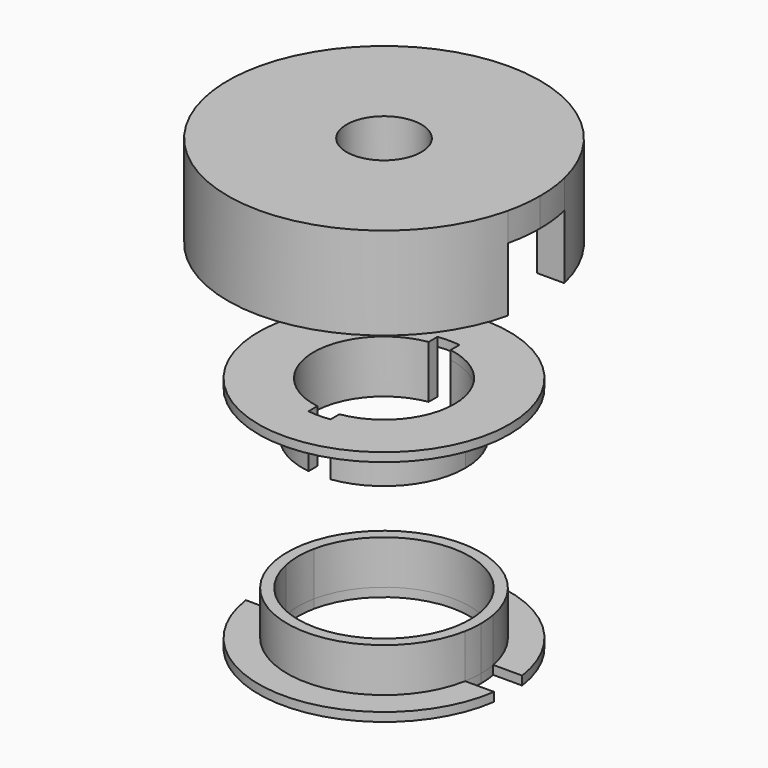
from build123d import *

# Parameters (mm, degrees)
F1_DEPTH  = 4.2
F0_R      = 3
F0_R_2    = 1.7
F2_DEPTH  = 1.3
F5_DEPTH  = 2
F4_R      = 5.7
F6_DEPTH  = 0.4
F7_DEPTH  = 2
F10_DEPTH = 2
F11_DEPTH = 0.4


with BuildPart() as f1:
    # F0 (on Top) → F1 (new body)
    with BuildSketch(Plane.XY):
        with BuildLine():
            Line((5.6789083458, 1.6), (6.9173694422, 1.6))
            ThreePointArc((6.9173694422, 1.6), (0, 7.1), (-6.9173694422, 1.6))
            Line((-6.9173694422, 1.6), (-5.6789083458, 1.6))
            ThreePointArc((-5.6789083458, 1.6), (0, 5.9), (5.6789083458, 1.6))
        make_face()
    extrude(amount=-F1_DEPTH)



with BuildPart() as f1b:
    # F0 (on Top) → F1, piece 2 (new body)
    with BuildSketch(Plane.XY):
        with BuildLine():
            ThreePointArc((-6.9173694422, -1.6), (0, -7.1), (6.9173694422, -1.6))
            Line((6.9173694422, -1.6), (5.6789083458, -1.6))
            ThreePointArc((5.6789083458, -1.6), (0, -5.9), (-5.6789083458, -1.6))
            Line((-5.6789083458, -1.6), (-6.9173694422, -1.6))
        make_face()
    extrude(amount=-F1_DEPTH)


with BuildPart() as f1c:
    # F0 (on Top) → F1, piece 3 (new body)
    with BuildSketch(Plane.XY):
        Circle(F0_R)
        Circle(F0_R_2, mode=Mode.SUBTRACT)
    extrude(amount=-F1_DEPTH)


with BuildPart() as f1_1:
    add(f1.part)

    add(f1b.part)  # F2 merges F1b

    add(f1c.part)  # F2 merges F1c
    # F0 (on Top) → F2 (join)
    with BuildSketch(Plane.XY):
        with BuildLine():
            Line((5.6789083458, 1.6), (6.9173694422, 1.6))
            ThreePointArc((6.9173694422, 1.6), (0, 7.1), (-6.9173694422, 1.6))
            Line((-6.9173694422, 1.6), (-5.6789083458, 1.6))
            ThreePointArc((-5.6789083458, 1.6), (0, 5.9), (5.6789083458, 1.6))
        make_face()
        with BuildLine():
            Line((-5.6789083458, 1.6), (-6.9173694422, 1.6))
            ThreePointArc((-6.9173694422, 1.6), (-7.1, 0), (-6.9173694422, -1.6))
            Line((-6.9173694422, -1.6), (-5.6789083458, -1.6))
            ThreePointArc((-5.6789083458, -1.6), (-5.9, 0), (-5.6789083458, 1.6))
        make_face()
        with BuildLine():
            ThreePointArc((-6.9173694422, -1.6), (0, -7.1), (6.9173694422, -1.6))
            Line((6.9173694422, -1.6), (5.6789083458, -1.6))
            ThreePointArc((5.6789083458, -1.6), (0, -5.9), (-5.6789083458, -1.6))
            Line((-5.6789083458, -1.6), (-6.9173694422, -1.6))
        make_face()
        with BuildLine():
            ThreePointArc((6.9173694422, -1.6), (7.0541946046, -0.8051946846), (7.1, 0))
            ThreePointArc((7.1, 0), (7.0541946046, 0.8051946846), (6.9173694422, 1.6))
            Line((6.9173694422, 1.6), (5.6789083458, 1.6))
            ThreePointArc((5.6789083458, 1.6), (5.8444657258, 0.807601622), (5.9, 0))
            ThreePointArc((5.9, 0), (5.8444657258, -0.807601622), (5.6789083458, -1.6))
            Line((5.6789083458, -1.6), (6.9173694422, -1.6))
        make_face()
        with BuildLine():
            Line((5.6789083458, -1.6), (5.6789083458, 1.6))
            ThreePointArc((5.6789083458, 1.6), (0, 5.9), (-5.6789083458, 1.6))
            Line((-5.6789083458, 1.6), (-5.6789083458, -1.6))
            ThreePointArc((-5.6789083458, -1.6), (0, -5.9), (5.6789083458, -1.6))
        make_face()
        Circle(F0_R, mode=Mode.SUBTRACT)
        with BuildLine():
            Line((-5.6789083458, -1.6), (-5.6789083458, 1.6))
            ThreePointArc((-5.6789083458, 1.6), (-5.9, 0), (-5.6789083458, -1.6))
        make_face()
        with BuildLine():
            ThreePointArc((5.9, 0), (5.8444657258, 0.807601622), (5.6789083458, 1.6))
            Line((5.6789083458, 1.6), (5.6789083458, -1.6))
            ThreePointArc((5.6789083458, -1.6), (5.8444657258, -0.807601622), (5.9, 0))
        make_face()
    extrude(amount=-F2_DEPTH)


with BuildPart() as f5:
    # F4 (on offset) → F5 (new body)
    with BuildSketch(Plane.XY.offset(-10)):
        with BuildLine():
            ThreePointArc((-0.5, 3.1606961259), (0, 3.2), (0.5, 3.1606961259))
            Line((0.5, 3.1606961259), (0.5, 3.666060556))
            ThreePointArc((0.5, 3.666060556), (0, 3.7), (-0.5, 3.666060556))
            Line((-0.5, 3.666060556), (-0.5, 3.1606961259))
        make_face()
        with BuildLine():
            ThreePointArc((-0.5, -3.1606961259), (-3.2, 0), (-0.5, 3.1606961259))
            Line((-0.5, 3.1606961259), (-0.5, 3.666060556))
            ThreePointArc((-0.5, 3.666060556), (-3.7, 0), (-0.5, -3.666060556))
            Line((-0.5, -3.666060556), (-0.5, -3.1606961259))
        make_face()
        with BuildLine():
            Line((0.5, -3.666060556), (0.5, -3.1606961259))
            ThreePointArc((0.5, -3.1606961259), (0, -3.2), (-0.5, -3.1606961259))
            Line((-0.5, -3.1606961259), (-0.5, -3.666060556))
            ThreePointArc((-0.5, -3.666060556), (0, -3.7), (0.5, -3.666060556))
        make_face()
        with BuildLine():
            ThreePointArc((0.5, 3.1606961259), (2.4331050121, 2.0784609691), (3.2, 0))
            ThreePointArc((3.2, 0), (2.4331050121, -2.0784609691), (0.5, -3.1606961259))
            Line((0.5, -3.1606961259), (0.5, -3.666060556))
            ThreePointArc((0.5, -3.666060556), (2.787471973, -2.4331050121), (3.7, 0))
            ThreePointArc((3.7, 0), (2.787471973, 2.4331050121), (0.5, 3.666060556))
            Line((0.5, 3.666060556), (0.5, 3.1606961259))
        make_face()
    extrude(amount=-F5_DEPTH)

    # F4 (on offset) → F6 (join)
    with BuildSketch(Plane.XY.offset(-10)):
        Circle(F4_R)
        with BuildLine():
            Line((0.5, 4.331942182), (0.5, 3.666060556))
            ThreePointArc((0.5, 3.666060556), (2.787471973, 2.4331050121), (3.7, 0))
            ThreePointArc((3.7, 0), (2.787471973, -2.4331050121), (0.5, -3.666060556))
            Line((0.5, -3.666060556), (0.5, -4.331942182))
            Line((0.5, -4.331942182), (-0.5, -4.331942182))
            Line((-0.5, -4.331942182), (-0.5, -3.666060556))
            ThreePointArc((-0.5, -3.666060556), (-3.7, 0), (-0.5, 3.666060556))
            Line((-0.5, 3.666060556), (-0.5, 4.331942182))
            Line((-0.5, 4.331942182), (0.5, 4.331942182))
        make_face(mode=Mode.SUBTRACT)
        with BuildLine():
            ThreePointArc((-0.5, -3.1606961259), (-3.2, 0), (-0.5, 3.1606961259))
            Line((-0.5, 3.1606961259), (-0.5, 3.666060556))
            ThreePointArc((-0.5, 3.666060556), (-3.7, 0), (-0.5, -3.666060556))
            Line((-0.5, -3.666060556), (-0.5, -3.1606961259))
        make_face()
        with BuildLine():
            ThreePointArc((0.5, 3.1606961259), (2.4331050121, 2.0784609691), (3.2, 0))
            ThreePointArc((3.2, 0), (2.4331050121, -2.0784609691), (0.5, -3.1606961259))
            Line((0.5, -3.1606961259), (0.5, -3.666060556))
            ThreePointArc((0.5, -3.666060556), (2.787471973, -2.4331050121), (3.7, 0))
            ThreePointArc((3.7, 0), (2.787471973, 2.4331050121), (0.5, 3.666060556))
            Line((0.5, 3.666060556), (0.5, 3.1606961259))
        make_face()
        with BuildLine():
            ThreePointArc((-0.5, 3.666060556), (0, 3.7), (0.5, 3.666060556))
            Line((0.5, 3.666060556), (0.5, 4.331942182))
            Line((0.5, 4.331942182), (-0.5, 4.331942182))
            Line((-0.5, 4.331942182), (-0.5, 3.666060556))
        make_face()
        with BuildLine():
            Line((0.5, -4.331942182), (0.5, -3.666060556))
            ThreePointArc((0.5, -3.666060556), (0, -3.7), (-0.5, -3.666060556))
            Line((-0.5, -3.666060556), (-0.5, -4.331942182))
            Line((-0.5, -4.331942182), (0.5, -4.331942182))
        make_face()
        with BuildLine():
            ThreePointArc((-0.5, 3.1606961259), (0, 3.2), (0.5, 3.1606961259))
            Line((0.5, 3.1606961259), (0.5, 3.666060556))
            ThreePointArc((0.5, 3.666060556), (0, 3.7), (-0.5, 3.666060556))
            Line((-0.5, 3.666060556), (-0.5, 3.1606961259))
        make_face()
        with BuildLine():
            Line((0.5, -3.666060556), (0.5, -3.1606961259))
            ThreePointArc((0.5, -3.1606961259), (0, -3.2), (-0.5, -3.1606961259))
            Line((-0.5, -3.1606961259), (-0.5, -3.666060556))
            ThreePointArc((-0.5, -3.666060556), (0, -3.7), (0.5, -3.666060556))
        make_face()
    extrude(amount=F6_DEPTH)

    # F4 (on offset) → F7 (cut, symmetric)
    with BuildSketch(Plane.XY.offset(-10)):
        with BuildLine():
            ThreePointArc((-0.5, 3.1606961259), (0, 3.2), (0.5, 3.1606961259))
            Line((0.5, 3.1606961259), (0.5, 3.666060556))
            ThreePointArc((0.5, 3.666060556), (0, 3.7), (-0.5, 3.666060556))
            Line((-0.5, 3.666060556), (-0.5, 3.1606961259))
        make_face()
        with BuildLine():
            Line((0.5, -3.666060556), (0.5, -3.1606961259))
            ThreePointArc((0.5, -3.1606961259), (0, -3.2), (-0.5, -3.1606961259))
            Line((-0.5, -3.1606961259), (-0.5, -3.666060556))
            ThreePointArc((-0.5, -3.666060556), (0, -3.7), (0.5, -3.666060556))
        make_face()
    extrude(amount=F7_DEPTH, both=True, mode=Mode.SUBTRACT)


with BuildPart() as f10:
    # F9 (on offset) → F10 (new body)
    with BuildSketch(Plane.XY.offset(-20)):
        with BuildLine():
            Line((3.8170669368, 0.8), (4.3266615306, 0.8))
            ThreePointArc((4.3266615306, 0.8), (0, 4.4), (-4.3266615306, 0.8))
            Line((-4.3266615306, 0.8), (-3.8170669368, 0.8))
            ThreePointArc((-3.8170669368, 0.8), (0, 3.9), (3.8170669368, 0.8))
        make_face()
        with BuildLine():
            Line((-3.8170669368, 0.8), (-4.3266615306, 0.8))
            ThreePointArc((-4.3266615306, 0.8), (-4.4, 0), (-4.3266615306, -0.8))
            Line((-4.3266615306, -0.8), (-3.8170669368, -0.8))
            ThreePointArc((-3.8170669368, -0.8), (-3.9, 0), (-3.8170669368, 0.8))
        make_face()
        with BuildLine():
            ThreePointArc((-4.3266615306, -0.8), (0, -4.4), (4.3266615306, -0.8))
            Line((4.3266615306, -0.8), (3.8170669368, -0.8))
            ThreePointArc((3.8170669368, -0.8), (0, -3.9), (-3.8170669368, -0.8))
            Line((-3.8170669368, -0.8), (-4.3266615306, -0.8))
        make_face()
        with BuildLine():
            ThreePointArc((4.4, 0), (4.3816270228, 0.4016772744), (4.3266615306, 0.8))
            Line((4.3266615306, 0.8), (3.8170669368, 0.8))
            ThreePointArc((3.8170669368, 0.8), (3.8792113279, 0.4021435978), (3.9, 0))
            ThreePointArc((3.9, 0), (3.8792113279, -0.4021435978), (3.8170669368, -0.8))
            Line((3.8170669368, -0.8), (4.3266615306, -0.8))
            ThreePointArc((4.3266615306, -0.8), (4.3816270228, -0.4016772744), (4.4, 0))
        make_face()
    extrude(amount=F10_DEPTH)

    # F9 (on offset) → F11 (join)
    with BuildSketch(Plane.XY.offset(-20)):
        with BuildLine():
            Line((4.3266615306, 0.8), (5.6435804238, 0.8))
            ThreePointArc((5.6435804238, 0.8), (0, 5.7), (-5.6435804238, 0.8))
            Line((-5.6435804238, 0.8), (-4.3266615306, 0.8))
            ThreePointArc((-4.3266615306, 0.8), (0, 4.4), (4.3266615306, 0.8))
        make_face()
        with BuildLine():
            ThreePointArc((-5.6435804238, -0.8), (0, -5.7), (5.6435804238, -0.8))
            Line((5.6435804238, -0.8), (4.3266615306, -0.8))
            ThreePointArc((4.3266615306, -0.8), (0, -4.4), (-4.3266615306, -0.8))
            Line((-4.3266615306, -0.8), (-5.6435804238, -0.8))
        make_face()
        with BuildLine():
            Line((3.8170669368, 0.8), (4.3266615306, 0.8))
            ThreePointArc((4.3266615306, 0.8), (0, 4.4), (-4.3266615306, 0.8))
            Line((-4.3266615306, 0.8), (-3.8170669368, 0.8))
            ThreePointArc((-3.8170669368, 0.8), (0, 3.9), (3.8170669368, 0.8))
        make_face()
        with BuildLine():
            ThreePointArc((4.4, 0), (4.3816270228, 0.4016772744), (4.3266615306, 0.8))
            Line((4.3266615306, 0.8), (3.8170669368, 0.8))
            ThreePointArc((3.8170669368, 0.8), (3.8792113279, 0.4021435978), (3.9, 0))
            ThreePointArc((3.9, 0), (3.8792113279, -0.4021435978), (3.8170669368, -0.8))
            Line((3.8170669368, -0.8), (4.3266615306, -0.8))
            ThreePointArc((4.3266615306, -0.8), (4.3816270228, -0.4016772744), (4.4, 0))
        make_face()
        with BuildLine():
            ThreePointArc((-4.3266615306, -0.8), (0, -4.4), (4.3266615306, -0.8))
            Line((4.3266615306, -0.8), (3.8170669368, -0.8))
            ThreePointArc((3.8170669368, -0.8), (0, -3.9), (-3.8170669368, -0.8))
            Line((-3.8170669368, -0.8), (-4.3266615306, -0.8))
        make_face()
        with BuildLine():
            Line((-3.8170669368, 0.8), (-4.3266615306, 0.8))
            ThreePointArc((-4.3266615306, 0.8), (-4.4, 0), (-4.3266615306, -0.8))
            Line((-4.3266615306, -0.8), (-3.8170669368, -0.8))
            ThreePointArc((-3.8170669368, -0.8), (-3.9, 0), (-3.8170669368, 0.8))
        make_face()
    extrude(amount=-F11_DEPTH)


solid = Compound([f1_1.part, f5.part, f10.part])
